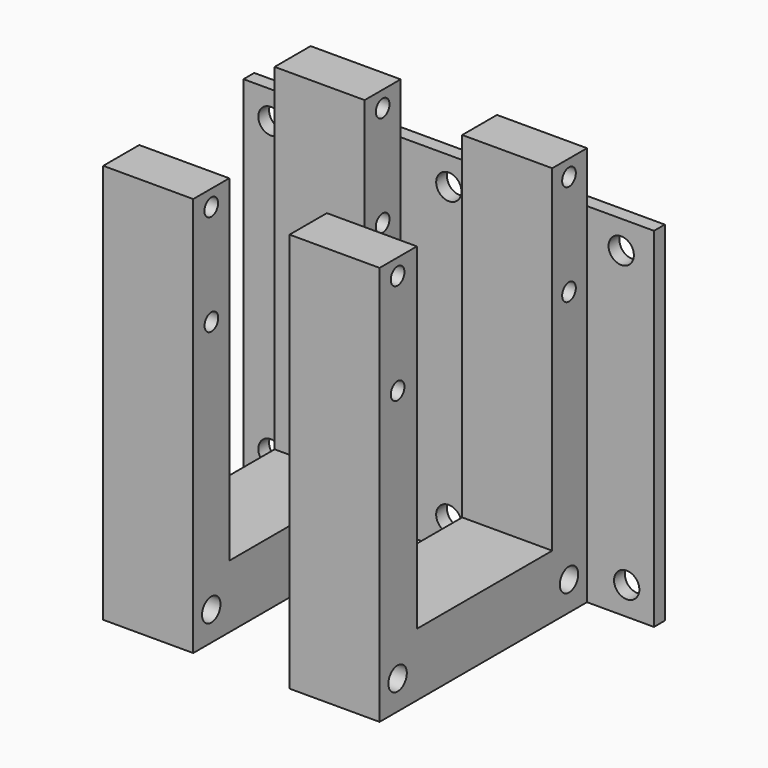
from build123d import *

# Parameters (mm, degrees)
F0_W     = 25.4
F0_H     = 14.3764
F0_H_2   = 98.3996
F1_DEPTH = 73.152
F0_W_2   = 27.178
F0_R     = 3.5687
F0_W_3   = 18.8976
F0_W_4   = 18.9484
F2_DEPTH = 3.81
F3_W     = 47.752
F3_H     = 94.996
F3_R     = 2.413
F3_R_2   = 3.2512
F4_DEPTH = 96.8766
F5_R     = 2.413
F5_R_2   = 3.2512
F5_W     = 47.7424701676
F5_H     = 94.996
F6_DEPTH = 25.4


with BuildPart() as f1:
    # F0 (on Front) → F1 (new body)
    with BuildSketch(Plane.XZ):
        with Locations((-23.7647381214, 45.8519933552)):
            Rectangle(F0_W, F0_H)
        with Locations((-23.7647381214, -10.5360066448)):
            Rectangle(F0_W, F0_H_2)
    extrude(amount=F1_DEPTH)

    # F3 (on face) → F4 (cut, through all)
    with BuildSketch(Plane(origin=(-36.4647381214, 0, 0), x_dir=(0, -1, 0), z_dir=(-1, 0, 0))):
        with Locations((36.576, 5.5421933552)):
            Rectangle(F3_W, F3_H)
        with Locations((6.35, 19.9439933552)):
            Circle(F3_R)
        with Locations((66.75198313, 19.9439933552)):
            Circle(F3_R)
        with Locations((66.802, 48.4681933552)):
            Circle(F3_R)
        with Locations((6.35, 48.4681933552)):
            Circle(F3_R)
        with Locations((6.35, -51.5062066448)):
            Circle(F3_R_2)
        with Locations((66.802, -51.5062066448)):
            Circle(F3_R_2)
    extrude(amount=-F4_DEPTH, mode=Mode.SUBTRACT)


with BuildPart() as f1b:
    # F0 (on Front) → F1, piece 2 (new body)
    with BuildSketch(Plane.XZ):
        with Locations((28.8132618786, -10.5360066448)):
            Rectangle(F0_W, F0_H_2)
        with Locations((28.8132618786, 45.8519933552)):
            Rectangle(F0_W, F0_H)
    extrude(amount=F1_DEPTH)

    # F5 (on face) → F6 (cut)
    with BuildSketch(Plane.YZ.offset(41.5132618786)):
        with Locations((-66.802, 48.4681933552)):
            Circle(F5_R)
        with Locations((-66.802, 19.9439933552)):
            Circle(F5_R)
        with Locations((-66.802, -51.5062066448)):
            Circle(F5_R_2)
        with Locations((-6.35, -51.5062066448)):
            Circle(F5_R_2)
        with Locations((-6.35, 19.9439933552)):
            Circle(F5_R)
        with Locations((-6.35, 48.4681933552)):
            Circle(F5_R)
        with Locations((-36.1322467215, 5.5421933552)):
            Rectangle(F5_W, F5_H)
    extrude(amount=-F6_DEPTH, mode=Mode.SUBTRACT)


with BuildPart() as f2:
    # F0 (on Front) → F2 (new body)
    with BuildSketch(Plane.XZ):
        with Locations((2.5242618786, -10.5360066448)):
            Rectangle(F0_W_2, F0_H_2)
        with Locations((2.5242618786, -51.8110066448)):
            Circle(F0_R, mode=Mode.SUBTRACT)
        with Locations((2.5242618786, 30.7389933552)):
            Circle(F0_R, mode=Mode.SUBTRACT)
        with Locations((50.9620618786, -10.5360066448)):
            Rectangle(F0_W_3, F0_H_2)
        with Locations((52.7146618786, -51.8110066448)):
            Circle(F0_R, mode=Mode.SUBTRACT)
        with Locations((51.1651380685, 30.7389933552)):
            Circle(F0_R, mode=Mode.SUBTRACT)
        with Locations((28.8132618786, -10.5360066448)):
            Rectangle(F0_W, F0_H_2)
        with Locations((-23.7647381214, -10.5360066448)):
            Rectangle(F0_W, F0_H_2)
        with Locations((-45.9389381214, -10.5360066448)):
            Rectangle(F0_W_4, F0_H_2)
        with Locations((-47.6661381214, -51.8110066448)):
            Circle(F0_R, mode=Mode.SUBTRACT)
        with Locations((-47.6661381214, 30.7389933552)):
            Circle(F0_R, mode=Mode.SUBTRACT)
    extrude(amount=-F2_DEPTH)


solid = Compound([f1.part, f1b.part, f2.part])
